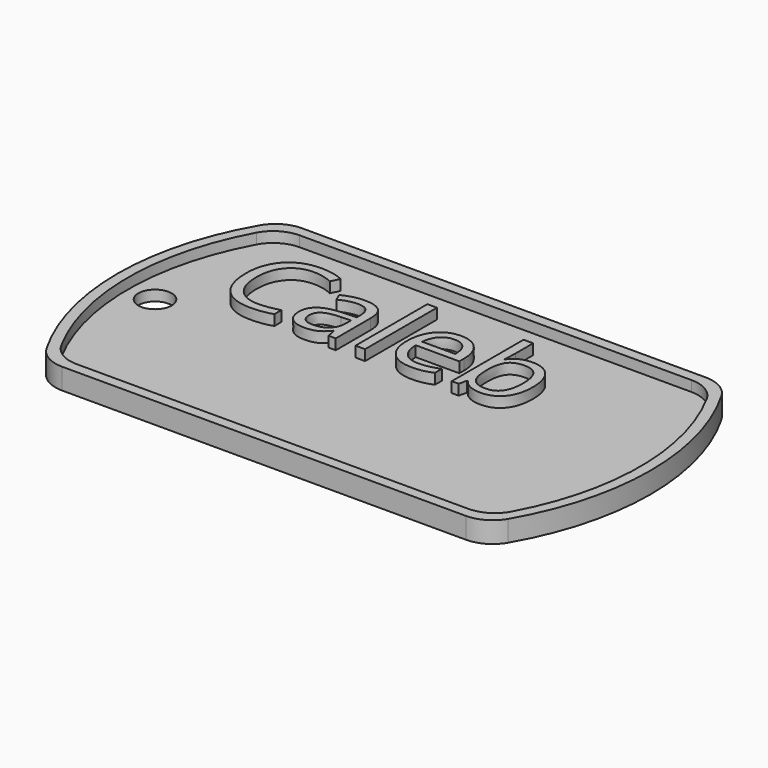
from build123d import *

# Parameters (mm, degrees)
F1_DEPTH     = 1
F3_DEPTH     = 1
F4_R         = 1.5875
F5_DEPTH     = 1
F6_TEXT_SIZE = 11.2669134269
F7_DEPTH     = 1


# Not quite as in the source:
# - Text() gives the source's letters only with a copy of the font that has no kerning and outlines rounded to 1/6400 em; it was checked with that copy


with BuildPart() as f1:
    # F0 (on Top) → F1 (new body)
    with BuildSketch(Plane.XY):
        with BuildLine():
            ThreePointArc((-19.2474145991, 14.2875), (-20.8349145991, 13.862130657), (-21.9970452561, 12.7))
            ThreePointArc((-21.9970452561, 12.7), (-25.4, 0), (-21.9970452561, -12.7))
            ThreePointArc((-21.9970452561, -12.7), (-20.8349145991, -13.862130657), (-19.2474145991, -14.2875))
            Line((-19.2474145991, -14.2875), (19.2474145991, -14.2875))
            ThreePointArc((19.2474145991, -14.2875), (20.8349145991, -13.862130657), (21.9970452561, -12.7))
            ThreePointArc((21.9970452561, -12.7), (25.4, 0), (21.9970452561, 12.7))
            ThreePointArc((21.9970452561, 12.7), (20.8349145991, 13.862130657), (19.2474145991, 14.2875))
            Line((19.2474145991, 14.2875), (-19.2474145991, 14.2875))
        make_face()
    extrude(amount=F1_DEPTH)

    # F2 (on face) → F3 (join)
    with BuildSketch(Plane.XY.offset(1)):
        with BuildLine():
            Line((19.2474145991, 14.2875), (-19.2474145991, 14.2875))
            ThreePointArc((-19.2474145991, 14.2875), (-20.8349145991, 13.862130657), (-21.9970452561, 12.7))
            ThreePointArc((-21.9970452561, 12.7), (-25.4, 0), (-21.9970452561, -12.7))
            ThreePointArc((-21.9970452561, -12.7), (-20.8349145991, -13.862130657), (-19.2474145991, -14.2875))
            Line((-19.2474145991, -14.2875), (19.2474145991, -14.2875))
            ThreePointArc((19.2474145991, -14.2875), (20.8349145991, -13.862130657), (21.9970452561, -12.7))
            ThreePointArc((21.9970452561, -12.7), (25.4, 0), (21.9970452561, 12.7))
            ThreePointArc((21.9970452561, 12.7), (20.8349145991, 13.862130657), (19.2474145991, 14.2875))
        make_face()
        with BuildLine():
            ThreePointArc((-21.4526124879, 11.6252061249), (-20.2856017842, 12.8404540819), (-18.6611352482, 13.2875))
            Line((-18.6611352482, 13.2875), (18.6611352482, 13.2875))
            ThreePointArc((18.6611352482, 13.2875), (20.2856017842, 12.8404540819), (21.4526124879, 11.6252061249))
            ThreePointArc((21.4526124879, 11.6252061249), (24.4, 0), (21.4526124879, -11.6252061249))
            ThreePointArc((21.4526124879, -11.6252061249), (20.2856017842, -12.8404540819), (18.6611352482, -13.2875))
            Line((18.6611352482, -13.2875), (-18.6611352482, -13.2875))
            ThreePointArc((-18.6611352482, -13.2875), (-20.2856017842, -12.8404540819), (-21.4526124879, -11.6252061249))
            ThreePointArc((-21.4526124879, -11.6252061249), (-24.4, 0), (-21.4526124879, 11.6252061249))
        make_face(mode=Mode.SUBTRACT)
    extrude(amount=F3_DEPTH)

    # F4 (on face) → F5 (cut)
    with BuildSketch(Plane.XY.offset(1)):
        with Locations((-21.821282804, 0)):
            Circle(F4_R)
    extrude(amount=-F5_DEPTH, mode=Mode.SUBTRACT)

    # F6 (on face) → F7 (join)
    with BuildSketch(Plane.XY.offset(1)):
        with Locations((-18.6611352482, 2.0003223326)):
            Text('Caleb', F6_TEXT_SIZE, font='Open Sans', text_align=(TextAlign.LEFT, TextAlign.BOTTOM))
    extrude(amount=F7_DEPTH)


solid = f1.part
